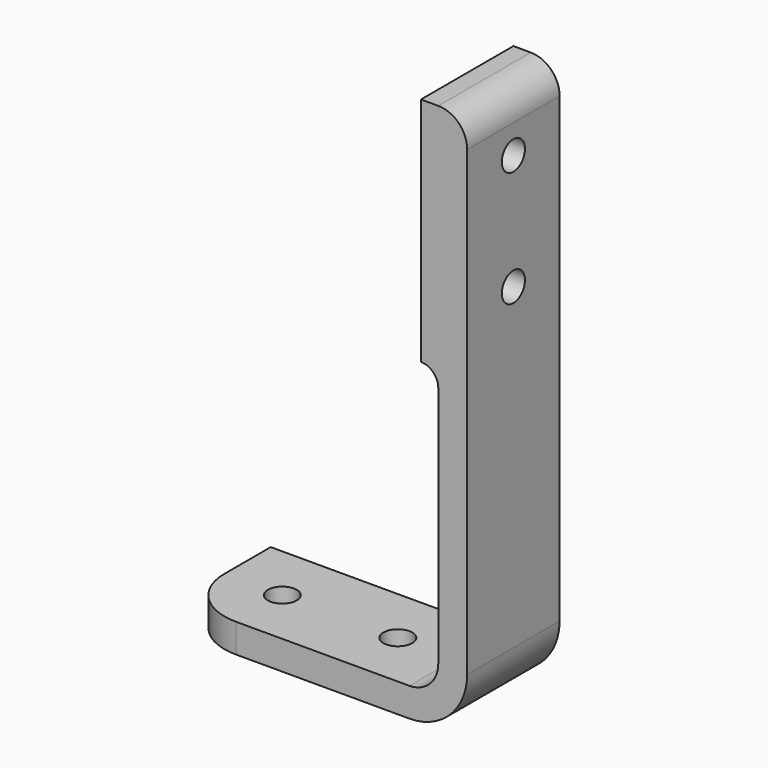
from build123d import *

# Parameters (mm, degrees)
F0_W     = 40
F0_H     = 5
F1_DEPTH = 20
F3_D     = 5
F5_D     = 5
F6_R     = 10


# Not quite as in the source:
# - a feature names something its author has since deleted; it is built from what else it names


with BuildPart() as f1:
    # F0 (on Front) → F1 (new body)
    with BuildSketch(Plane.XZ):
        Polygon((19.9351918133, 52), (19.9351918133, 10), (24.9351918133, 10), (24.9351918133, 90), (19.9351918133, 90), (19.9351918133, 55), align=None)
        with Locations((-5.0648081867, 2.5)):
            Rectangle(F0_W, F0_H)
        with BuildLine():
            ThreePointArc((19.9351918133, 10), (18.4707257193, 6.4644660941), (14.9351918133, 5))
            Line((14.9351918133, 5), (14.9351918133, 0))
            ThreePointArc((14.9351918133, 0), (22.0062596252, 2.9289321881), (24.9351918133, 10))
            Line((24.9351918133, 10), (19.9351918133, 10))
        make_face()
        Polygon((16.9351918133, 55), (19.9351918133, 55), (19.9351918133, 90), (19.9351918133, 95), (16.9351918133, 95), align=None)
        with BuildLine():
            Line((19.9351918133, 90), (24.9351918133, 90))
            ThreePointArc((24.9351918133, 90), (23.4707257193, 93.5355339059), (19.9351918133, 95))
            Line((19.9351918133, 95), (19.9351918133, 90))
        make_face()
        with BuildLine():
            ThreePointArc((16.9351918133, 55), (19.0565121569, 54.1213203436), (19.9351918133, 52))
            Line((19.9351918133, 52), (19.9351918133, 55))
            Line((19.9351918133, 55), (16.9351918133, 55))
        make_face()
    extrude(amount=F1_DEPTH)

    # F3 (through all)
    with Locations(Plane(origin=(0, 0, 0), x_dir=(0, 1, 0), z_dir=(-1, 0, 0))):
        with Locations((-10, -85), (-10, -65)):
            Hole(F3_D / 2)

    # F5 (through all)
    with Locations(Plane(origin=(0, 0, 0), x_dir=(1, 0, 0), z_dir=(0, 0, -1))):
        with Locations((-15.0648081867, 10), (4.9351918133, 10)):
            Hole(F5_D / 2)

    # F6
    f6_edges = [f1.edges().sort_by_distance(p)[0] for p in [
        (-25.064808, -20, 2.5),
    ]]
    fillet(f6_edges, radius=F6_R)


solid = f1.part
